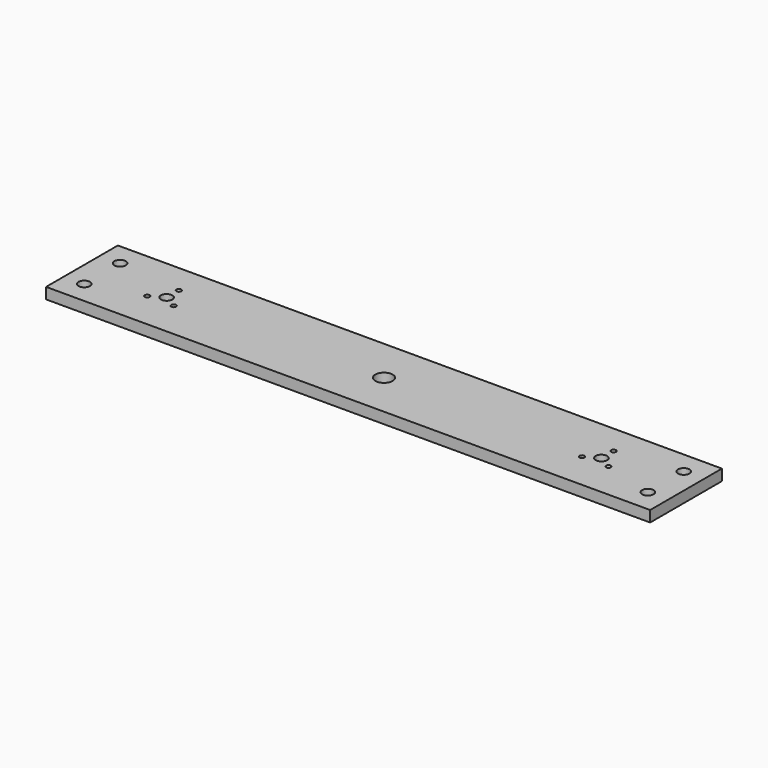
from build123d import *

# Parameters (mm, degrees)
F0_W     = 347.3
F0_H     = 51.58
F0_R     = 3.3
F0_R_2   = 5
F1_DEPTH = 6.35
F3_D     = 6.6
F4_R     = 1.4
F5_DEPTH = 6.351


# Not quite as in the source:
# - a feature names something its author has since deleted; it is built from what else it names


with BuildPart() as f1:
    # F0 (on Top) → F1 (new body)
    with BuildSketch(Plane.XY):
        Rectangle(F0_W, F0_H)
        with Locations((-125, 0)):
            Circle(F0_R, mode=Mode.SUBTRACT)
        Circle(F0_R_2, mode=Mode.SUBTRACT)
        with Locations((125, 0)):
            Circle(F0_R, mode=Mode.SUBTRACT)
    extrude(amount=F1_DEPTH)

    # F3 (through all)
    with Locations(Plane(origin=(0, 0, 0), x_dir=(1, 0, 0), z_dir=(0, 0, -1))):
        with Locations((-162.023125, 12.895), (-162.023125, -12.895), (162.023125, -12.895), (162.023125, 12.895)):
            Hole(F3_D / 2)

    # F4 (on face) → F5 (cut, through all)
    with BuildSketch(Plane.XY.offset(6.35)):
        with Locations((-125, 8.78)):
            Circle(F4_R)
        with Locations((-132.6037030452, -4.39)):
            Circle(F4_R)
        with Locations((-117.3962969548, -4.39)):
            Circle(F4_R)
        with Locations((125, 8.78)):
            Circle(F4_R)
        with Locations((132.6037030452, -4.39)):
            Circle(F4_R)
        with Locations((117.3962969548, -4.39)):
            Circle(F4_R)
    extrude(amount=-F5_DEPTH, mode=Mode.SUBTRACT)


solid = f1.part
